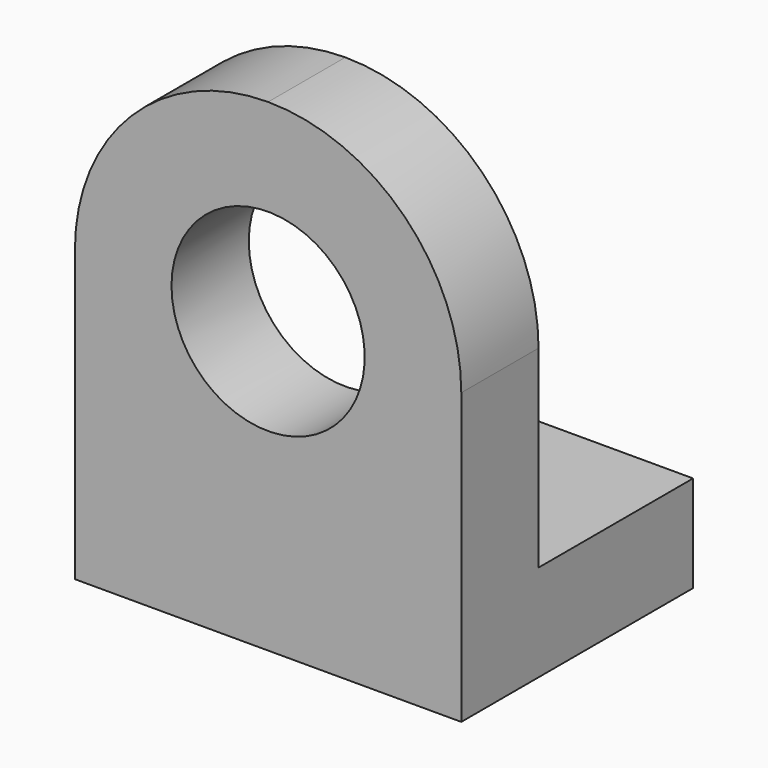
from build123d import *

# Parameters (mm, degrees)
F0_W     = 50.8
F0_H     = 38.1
F1_DEPTH = 12.7
F2_W     = 50.8
F2_H     = 12.7
F3_DEPTH = 63.5
F4_W     = 12.7
F4_H     = 12.7
F5_DEPTH = 12.701
F6_R     = 12.7
F7_DEPTH = 12.701
F8_R     = 25.39999


# Not quite as in the source:
# - a fillet or chamfer is up to 0.001 mm smaller than in the source, because OpenCascade refuses the exact size


with BuildPart() as f1:
    # F0 (on Top) → F1 (new body)
    with BuildSketch(Plane.XY):
        with Locations((-25.4, 19.05)):
            Rectangle(F0_W, F0_H)
    extrude(amount=F1_DEPTH)

    # F2 (on face) → F3 (join)
    with BuildSketch(Plane(origin=(0, 0, 0), x_dir=(1, 0, 0), z_dir=(0, 0, -1))):
        with Locations((-25.4, -6.35)):
            Rectangle(F2_W, F2_H)
    extrude(amount=-F3_DEPTH)

    # F4 (on face) → F5 (cut, through all)
    with BuildSketch(Plane.XY.offset(12.7)):
        with Locations((-44.45, 31.75)):
            Rectangle(F4_W, F4_H)
    extrude(amount=-F5_DEPTH, mode=Mode.SUBTRACT)

    # F6 (on face) → F7 (cut, through all)
    with BuildSketch(Plane(origin=(0, 12.7, 0), x_dir=(-1, 0, 0), z_dir=(0, 1, 0))):
        with Locations((25.4, 38.1)):
            Circle(F6_R)
    extrude(amount=-F7_DEPTH, mode=Mode.SUBTRACT)

    # F8 (radius 25.4 in the source; OpenCascade refuses exactly that, so slightly less here)
    f8_edges = [f1.edges().sort_by_distance(p)[0] for p in [
        (-50.8, 6.35, 63.5),
        (0, 6.35, 63.5),
    ]]
    fillet(f8_edges, radius=F8_R)


solid = f1.part
